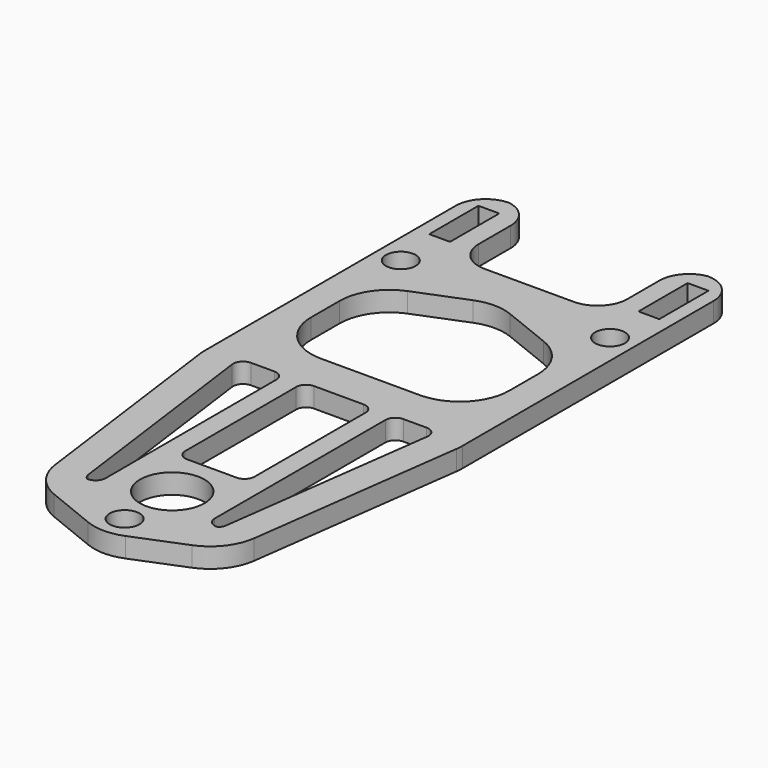
from build123d import *

# Parameters (mm, degrees)
F0_R         = 1.5
F0_W         = 2.1
F0_H         = 6.2
F1_DEPTH     = 2
F2_R         = 3
F4_DEPTH     = 2.001
F5_R         = 5
F6_T1_DEPTH  = 16.7901994578
F7_W         = 7
F7_H         = 16
F7_R         = 3.25
F8_DEPTH     = 2.001
F9_R         = 5
F10_T1_DEPTH = 2


# Not quite as in the source:
# - a fillet or chamfer that OpenCascade refuses, or shapes differently, is made with other operations: its cross-section is extruded or revolved along the edge and cut away or added


with BuildPart() as f1:
    # F0 (on Top) → F1 (new body)
    with BuildSketch(Plane.XY):
        Polygon((-13, -32), (13, -32), (13, 32), (7.5, 32), (7.5, 22), (-7.5, 22), (-7.5, 32), (-13, 32), align=None)
        with Locations((0, -29)):
            Circle(F0_R, mode=Mode.SUBTRACT)
        with Locations((-10.55, 19)):
            Circle(F0_R, mode=Mode.SUBTRACT)
        with Locations((-10.55, 27)):
            Rectangle(F0_W, F0_H, mode=Mode.SUBTRACT)
        with Locations((10.55, 19)):
            Circle(F0_R, mode=Mode.SUBTRACT)
        with Locations((10.55, 27)):
            Rectangle(F0_W, F0_H, mode=Mode.SUBTRACT)
    extrude(amount=F1_DEPTH)

    # F2
    f2_edges = [f1.edges().sort_by_distance(p)[0] for p in [
        (13, 32, 1),
        (7.5, 22, 1),
        (-7.5, 22, 1),
        (-13, 32, 1),
    ]]
    fillet(f2_edges, radius=F2_R)

    # F3 (on face) → F4 (cut, through all)
    with BuildSketch(Plane.XY.offset(2)):
        Polygon((-9.65, -28.1011469207), (-13, -3), (-13, -33), (13, -33), (13, -3), (9.65, -28.1011469207), (0, -32), align=None)
    extrude(amount=-F4_DEPTH, mode=Mode.SUBTRACT)

    # F5
    f5_edges = [f1.edges().sort_by_distance(p)[0] for p in [
        (9.65, -28.101147, 1),
        (-9.65, -28.101147, 1),
        (13, -3, 1),
        (0, -32, 1),
        (-13, -3, 1),
    ]]
    fillet(f5_edges, radius=F5_R)

    # F6: fillet of radius 3 on 2 edges, made by hand

    # F6_s2 → F6_t1 (cut)
    with BuildSketch(Plane.XY.offset(-7.3950997289)):
        with BuildLine():
            ThreePointArc((-7.5, 29.0419601084), (-8.2087121525, 30.9784517816), (-10, 32))
            Line((-10, 32), (-7.5, 32))
            Line((-7.5, 32), (-7.5, 29.0419601084))
        make_face()
        with BuildLine():
            ThreePointArc((10, 32), (8.2087121525, 30.9784517816), (7.5, 29.0419601084))
            Line((7.5, 29.0419601084), (7.5, 32))
            Line((7.5, 32), (10, 32))
        make_face()
    extrude(amount=F6_T1_DEPTH, mode=Mode.SUBTRACT)

    # F7 (on face) → F8 (cut, through all)
    with BuildSketch(Plane.XY.offset(2)):
        Polygon((10, 14), (0, 18), (-10, 14), (-10, 2), (10, 2), align=None)
        Polygon((-5.5, -2), (-10, -2), (-6.8708787487, -25.4461290331), (-5.5, -26), align=None)
        Polygon((6.8708787487, -25.4461290331), (10, -2), (5.5, -2), (5.5, -26), align=None)
        with Locations((0, -10)):
            Rectangle(F7_W, F7_H)
        with Locations((0, -23)):
            Circle(F7_R)
    extrude(amount=-F8_DEPTH, mode=Mode.SUBTRACT)

    # F9
    f9_edges = [f1.edges().sort_by_distance(p)[0] for p in [
        (-10, 14, 1),
        (0, 18, 1),
        (10, 14, 1),
        (-10, 2, 1),
        (10, 2, 1),
    ]]
    fillet(f9_edges, radius=F9_R)

    # F10: fillet of radius 1 on 12 edges, made by hand

    # F10_s2 → F10_t1 (join)
    with BuildSketch(Plane.XY):
        with BuildLine():
            ThreePointArc((-8.8576734794, -2), (-9.6100985971, -2.3413222015), (-9.8488849195, -3.1322871156))
            Line((-9.8488849195, -3.1322871156), (-10, -2))
            Line((-10, -2), (-8.8576734794, -2))
        make_face()
        with BuildLine():
            ThreePointArc((-3.5, -3), (-3.2071067812, -2.2928932188), (-2.5, -2))
            Line((-2.5, -2), (-3.5, -2))
            Line((-3.5, -2), (-3.5, -3))
        make_face()
        with BuildLine():
            ThreePointArc((6.5, -2), (5.7928932188, -2.2928932188), (5.5, -3))
            Line((5.5, -3), (5.5, -2))
            Line((5.5, -2), (6.5, -2))
        make_face()
        with BuildLine():
            ThreePointArc((-5.5, -3), (-5.7928932188, -2.2928932188), (-6.5, -2))
            Line((-6.5, -2), (-5.5, -2))
            Line((-5.5, -2), (-5.5, -3))
        make_face()
        with BuildLine():
            ThreePointArc((3.5, -3), (3.2071067812, -2.2928932188), (2.5, -2))
            Line((2.5, -2), (3.5, -2))
            Line((3.5, -2), (3.5, -3))
        make_face()
        with BuildLine():
            ThreePointArc((9.8488849195, -3.1322871156), (9.6100985971, -2.3413222015), (8.8576734794, -2))
            Line((8.8576734794, -2), (10, -2))
            Line((10, -2), (9.8488849195, -3.1322871156))
        make_face()
        with BuildLine():
            ThreePointArc((-3.5, -17), (-3.2071067812, -17.7071067812), (-2.5, -18))
            Line((-2.5, -18), (-3.5, -18))
            Line((-3.5, -18), (-3.5, -17))
        make_face()
        with BuildLine():
            ThreePointArc((2.5, -18), (3.2071067812, -17.7071067812), (3.5, -17))
            Line((3.5, -17), (3.5, -18))
            Line((3.5, -18), (2.5, -18))
        make_face()
        with BuildLine():
            ThreePointArc((-6.3312640971, -25.6641475042), (-6.7468030166, -25.3498829497), (-6.9478689438, -24.8692507652))
            Line((-6.9478689438, -24.8692507652), (-6.8708787487, -25.4461290331))
            Line((-6.8708787487, -25.4461290331), (-6.3312640971, -25.6641475042))
        make_face()
        with BuildLine():
            ThreePointArc((6.9478689438, -24.8692507652), (6.7468030166, -25.3498829497), (6.3312640971, -25.6641475042))
            Line((6.3312640971, -25.6641475042), (6.8708787487, -25.4461290331))
            Line((6.8708787487, -25.4461290331), (6.9478689438, -24.8692507652))
        make_face()
        with BuildLine():
            ThreePointArc((5.5, -24.5174390315), (5.9408070965, -25.346476604), (6.8746065934, -25.4446228861))
            Line((6.8746065934, -25.4446228861), (5.5, -26))
            Line((5.5, -26), (5.5, -24.5174390315))
        make_face()
        with BuildLine():
            ThreePointArc((-6.8746065934, -25.4446228861), (-5.9408070965, -25.346476604), (-5.5, -24.5174390315))
            Line((-5.5, -24.5174390315), (-5.5, -26))
            Line((-5.5, -26), (-6.8746065934, -25.4446228861))
        make_face()
    extrude(amount=F10_T1_DEPTH)


solid = f1.part
